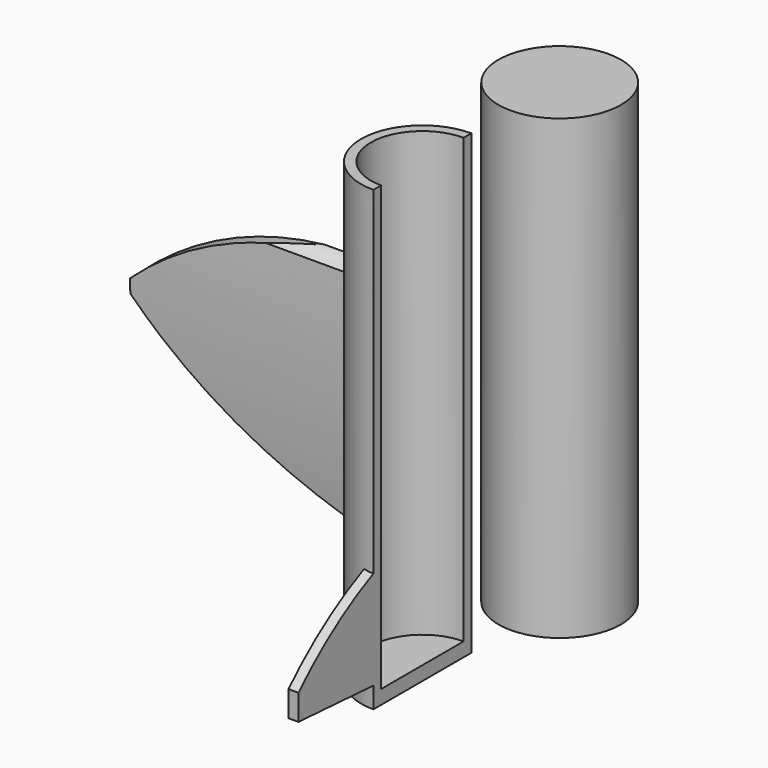
from build123d import *

# Parameters (mm, degrees)
F2_R          = 15.5434576405
F3_DEPTH      = 116.078
F5_DEPTH      = 2.54
F5_DEPTH_BACK = 2.54
F7_DEPTH      = 76.2
F7_DEPTH_BACK = 76.2
F9_DEPTH      = 72.898
F11_DEPTH     = 25.4
F12_R         = 13.0839369501
F13_DEPTH     = 112.522
F14_W         = 116.2168830633
F14_H         = 197.326593101
F15_DEPTH     = 105.156
F16_R         = 15.5448
F17_DEPTH     = 116.078


# Not quite as in the source:
# - the program builds the solid bodies; features that only make, move or delete a surface that nothing else refers to are left out


with BuildPart() as f3:
    # F2 (on face) → F3 (new body)
    with BuildSketch(Plane(origin=(0, 0, 0), x_dir=(1, 0, 0), z_dir=(0, 0, -1))):
        Circle(F2_R)
    extrude(amount=F3_DEPTH)

    # F4 (on Right) → F5 (join, two sides)
    with BuildSketch(Plane.YZ) as f5_sk:
        with BuildLine():
            Line((-11.3897956908, -111.0316067934), (-11.3897956908, -83.9041918516))
            ThreePointArc((-11.3897956908, -83.9041918516), (-26.3259256593, -91.8493771932), (-39.3006689847, -102.7061715722))
            Line((-39.3006689847, -102.7061715722), (-39.3006689847, -109.2196330428))
            Line((-39.3006689847, -109.2196330428), (-11.3897956908, -111.0316067934))
        make_face()
    extrude(amount=F5_DEPTH)
    extrude(f5_sk.sketch, amount=-F5_DEPTH_BACK)

    # F6 (on Right) → F7 (join, two sides)
    with BuildSketch(Plane.YZ) as f7_sk:
        with BuildLine():
            Line((5.9235603549, -91.6656255722), (5.9235603549, -30.5577199906))
            ThreePointArc((5.9235603549, -30.5577199906), (4.051450151, -31.3912602494), (2.6208171621, -32.8585281968))
            ThreePointArc((2.6208171621, -32.8585281968), (2.92151535, -62.3379338406), (5.9235603549, -91.6656255722))
        make_face()
    extrude(amount=F7_DEPTH)
    extrude(f7_sk.sketch, amount=-F7_DEPTH_BACK)

    # F8 (on Front) → F9 (cut)
    with BuildSketch(Plane.XZ):
        with BuildLine():
            ThreePointArc((-81.6321894526, -57.4373714626), (-51.7546829498, -36.2353974331), (-15.6106846407, -30.2520468831))
            Line((-15.6106846407, -30.2520468831), (-81.6321894526, -24.7040204704))
            Line((-81.6321894526, -24.7040204704), (-81.6321894526, -57.4373714626))
        make_face()
    extrude(amount=-F9_DEPTH, mode=Mode.SUBTRACT)

    # F10 (on Front) → F11 (cut)
    with BuildSketch(Plane.XZ):
        with BuildLine():
            ThreePointArc((-16.4980906993, -91.8035656214), (-49.0002384885, -77.3256808029), (-76.6182541847, -54.8925809562))
            Line((-76.6182541847, -54.8925809562), (-93.9552336931, -110.2590560913))
            Line((-93.9552336931, -110.2590560913), (-16.4980906993, -91.8035656214))
        make_face()
    extrude(amount=-F11_DEPTH, mode=Mode.SUBTRACT)

    # F12 (on Top) → F13 (cut)
    with BuildSketch(Plane.XY):
        Circle(F12_R)
    extrude(amount=-F13_DEPTH, mode=Mode.SUBTRACT)

    # F14 (on Right) → F15 (cut)
    with BuildSketch(Plane.YZ):
        with Locations((-3.3746473491, -56.032512337)):
            Rectangle(F14_W, F14_H)
    extrude(amount=F15_DEPTH, mode=Mode.SUBTRACT)


with BuildPart() as f17:
    # F16 (on Top) → F17 (new body)
    with BuildSketch(Plane.XY):
        with Locations((0, 43.5636749731)):
            Circle(F16_R)
    extrude(amount=-F17_DEPTH)


solid = Compound([f3.part, f17.part])
